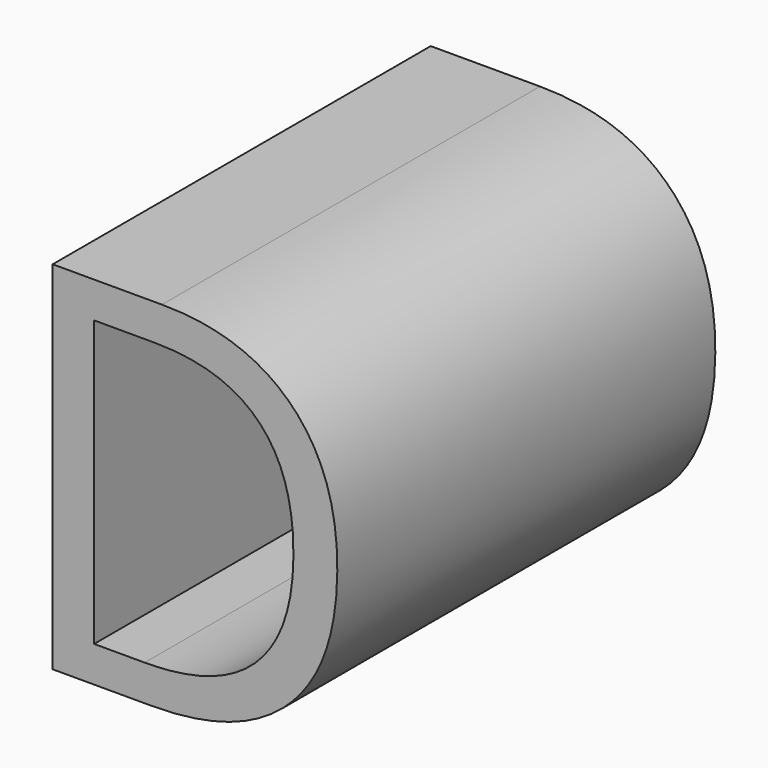
from build123d import *

# Parameters (mm, degrees)
F0_TEXT_SIZE = 104.7059479687
F2_DEPTH     = 99.0509614348


# Not quite as in the source:
# - Text() gives the source's letters only with a copy of the font that has no kerning and outlines rounded to 1/6400 em; it was checked with that copy


with BuildPart() as f2:
    # F0 (on Front) → F2 (new body)
    with BuildSketch(Plane.XZ):
        with Locations((0, 0)):
            Text('D', F0_TEXT_SIZE, font='Open Sans', text_align=(TextAlign.LEFT, TextAlign.BOTTOM))
    extrude(amount=-F2_DEPTH)


solid = f2.part
